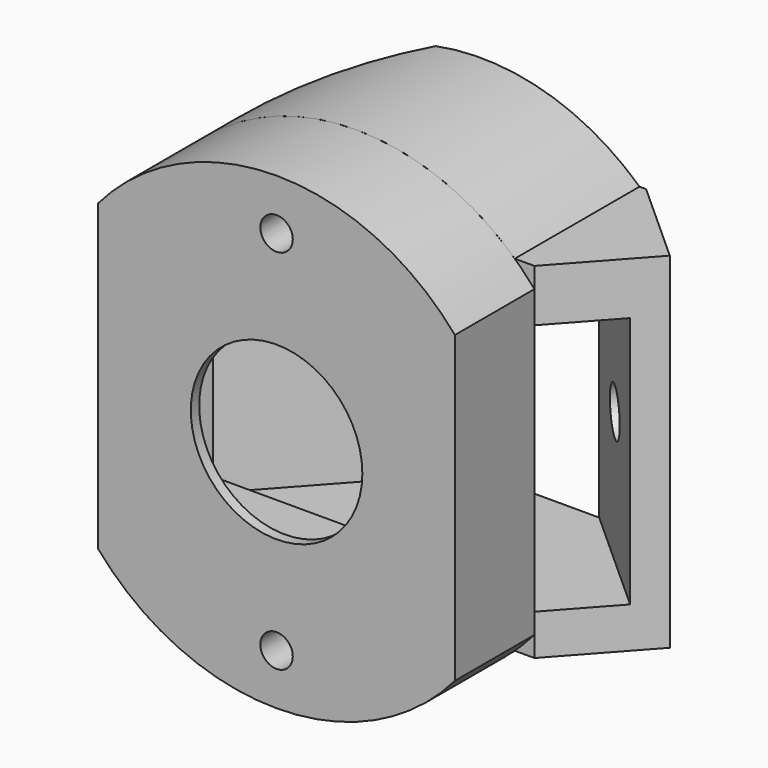
from build123d import *

# Parameters (mm, degrees)
F2_W           = 34.1
F2_H           = 29.1
F2_W_2         = 30.3
F2_H_2         = 25.3
F3_DEPTH       = 7.5
F3_DEPTH_BACK  = 1
F4_W           = 34.1
F4_H           = 29.1
F4_R           = 8.2
F5_DEPTH       = 1
F6_W           = 30.3
F6_H           = 25.3
F6_W_2         = 28.3
F6_H_2         = 21.1
F7_DEPTH       = 7.5
F9_DEPTH       = 8.5
F9_DEPTH_BACK  = 1
F10_R          = 1.55
F11_DEPTH      = 1.001
F11_DEPTH_BACK = 8.501
F12_R          = 2.5
F13_DEPTH      = 25
F14_R          = 0.8
F15_DEPTH      = 7.5
F18_DEPTH      = 22.5
F20_DEPTH      = 12.6
F20_DEPTH_BACK = 11.5
F21_R          = 2.25
F22_DEPTH      = 8.4193905153
F23_R          = 1.25
F24_DEPTH      = 15.9017858469
F26_DEPTH      = 15.9017858469


# Not quite as in the source:
# - a pattern or mirror of a feature is missing from the dataset's text; its kind, count and spacing are read off the source's solid


with BuildPart() as f3:
    # F2 (on Front) → F3 (new body, two sides)
    with BuildSketch(Plane.XZ) as f3_sk:
        Rectangle(F2_W, F2_H)
        Rectangle(F2_W_2, F2_H_2, mode=Mode.SUBTRACT)
    extrude(amount=F3_DEPTH)
    extrude(f3_sk.sketch, amount=-F3_DEPTH_BACK)

    # F4 (on face) → F5 (join)
    with BuildSketch(Plane.XZ.offset(7.5)):
        Rectangle(F4_W, F4_H)
        Circle(F4_R, mode=Mode.SUBTRACT)
    extrude(amount=F5_DEPTH)

    # F6 (on Front) → F7 (join, through all)
    with BuildSketch(Plane.XZ):
        Rectangle(F6_W, F6_H)
        Rectangle(F6_W_2, F6_H_2, mode=Mode.SUBTRACT)
    extrude(amount=F7_DEPTH)

    # F8 (on Front) → F9 (join, two sides)
    with BuildSketch(Plane.XZ) as f9_sk:
        with BuildLine():
            ThreePointArc((17.05, 14.55), (0, 22.4143926976), (-17.05, 14.55))
            Line((-17.05, 14.55), (17.05, 14.55))
        make_face()
        with BuildLine():
            ThreePointArc((-17.05, -14.55), (0, -22.4143926976), (17.05, -14.55))
            Line((17.05, -14.55), (-17.05, -14.55))
        make_face()
    extrude(amount=F9_DEPTH)
    extrude(f9_sk.sketch, amount=-F9_DEPTH_BACK)

    # F10 (on Front) → F11 (cut, two sides)
    with BuildSketch(Plane.XZ) as f11_sk:
        with Locations((0, 17.55)):
            Circle(F10_R)
        with Locations((0, -17.55)):
            Circle(F10_R)
    extrude(amount=-F11_DEPTH, mode=Mode.SUBTRACT)
    extrude(f11_sk.sketch, amount=F11_DEPTH_BACK, mode=Mode.SUBTRACT)

    # F12 (on face) → F13 (cut)
    with BuildSketch(Plane.XZ):
        with Locations((12.15, 12.55)):
            Circle(F12_R)
        with Locations((-12.15, 12.55)):
            Circle(F12_R)
        with Locations((-12.15, -12.55)):
            Circle(F12_R)
        with Locations((12.15, -12.55)):
            Circle(F12_R)
    extrude(amount=-F13_DEPTH, mode=Mode.SUBTRACT)

    # F14 (on Front) → F15 (cut, through all)
    with BuildSketch(Plane.XZ):
        with Locations((12.15, 12.55)):
            Circle(F14_R)
        with Locations((-12.15, 12.55)):
            Circle(F14_R)
        with Locations((-12.15, -12.55)):
            Circle(F14_R)
        with Locations((12.15, -12.55)):
            Circle(F14_R)
    extrude(amount=F15_DEPTH, mode=Mode.SUBTRACT)


with BuildPart() as f18:
    # F17 (on Top) → F18 (new body, symmetric)
    with BuildSketch(Plane.XY):
        Polygon((15.8040770662, 15.9007858469), (-4.3060885251, 15.9007858469), (-17.05, 1.7472382749), (-17.05, 1), (17.05, 1), (23.9017346294, 8.6096222277), align=None)
    extrude(amount=F18_DEPTH, both=True)

    # F19 (on Top) → F20 (cut, two sides)
    with BuildSketch(Plane.XY) as f20_sk:
        Polygon((-14.5863222203, 0), (28.9802591738, 0), (11.3206474166, 15.9007858469), (-0.2691903362, 15.9007858469), align=None)
        Polygon((-14.8685498887, -0.3134455806), (-14.5863222203, 0), (-15.2166664732, 0), align=None)
    extrude(amount=-F20_DEPTH, mode=Mode.SUBTRACT)
    extrude(f20_sk.sketch, amount=F20_DEPTH_BACK, mode=Mode.SUBTRACT)

    # F21 (on face) → F22 (cut, through all)
    with BuildSketch(Plane(origin=(12.9754986086, 14.4107511409, 0), x_dir=(0.7431448255, -0.6691306064, 0), z_dir=(-0.6691306064, -0.7431448255, 0))):
        with Locations((4.9602501193, 0)):
            Circle(F21_R)
    extrude(amount=-F22_DEPTH, mode=Mode.SUBTRACT)

    # F23 (on Front) → F24 (cut, through all)
    with BuildSketch(Plane.XZ):
        with Locations((0, 17.5)):
            Circle(F23_R)
        with Locations((0, -17.5)):
            Circle(F23_R)
    extrude(amount=-F24_DEPTH, mode=Mode.SUBTRACT)

    # F25 (on Front) → F26 (cut, through all)
    with BuildSketch(Plane.XZ):
        with BuildLine():
            Line((-20.9939805572, 29.1438214481), (-20.9939805572, 7.8522468355))
            ThreePointArc((-20.9939805572, 7.8522468355), (-5.2127815316, 21.799814419), (15.1708602261, 16.5))
            Line((15.1708602261, 16.5), (34.9690280855, 16.5))
            Line((34.9690280855, 16.5), (34.9690280855, 29.1438214481))
            Line((34.9690280855, 29.1438214481), (-20.9939805572, 29.1438214481))
        make_face()
    f26 = extrude(amount=-F26_DEPTH, mode=Mode.SUBTRACT)

    # F26_copies: F26 across plane
    add(f26.mirror(Plane(origin=(0, 0, 0), x_dir=(-1, 0, 0), z_dir=(0, 0, -1))), mode=Mode.SUBTRACT)


solid = Compound([f3.part, f18.part])
